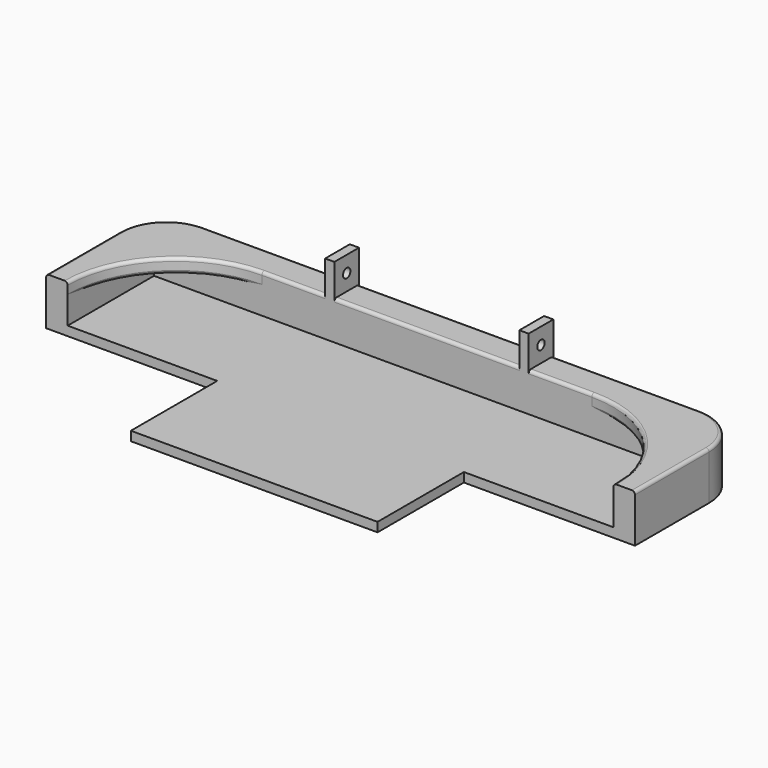
from build123d import *

# Parameters (mm, degrees)
F0_W         = 80
F0_H         = 35
F0_W_2       = 60
F0_H_2       = 10
F0_W_3       = 3
F1_DEPTH     = 3
F2_DEPTH     = 12.525
F3_DEPTH     = 7.968
F4_DEPTH     = 23
F5_R         = 1.5
F6_DEPTH     = 128.501
F7_T1_DEPTH  = 60
F7_T3_DEPTH  = 47.5
F7_T5_DEPTH  = 20.5
F7_T7_DEPTH  = 32.5
F7_T9_DEPTH  = 20.5
F7_T11_DEPTH = 47.5
F7_T16_ANGLE = 130.941996925
F7_T22_ANGLE = 130.941996925
F7_T26_ANGLE = 94.0941996925
F7_T28_ANGLE = 94.0941996925
F7_T30_ANGLE = 90
F7_T32_ANGLE = 90


# Not quite as in the source:
# - a fillet or chamfer that OpenCascade refuses, or shapes differently, is made with other operations: its cross-section is extruded or revolved along the edge and cut away or added


with BuildPart() as f1:
    # F0 (on Top) → F1 (new body)
    with BuildSketch(Plane.XY):
        with Locations((0, -17.5)):
            Rectangle(F0_W, F0_H)
        with BuildLine():
            Line((-88.5, 35), (-88.5, 0))
            ThreePointArc((-88.5, 0), (-78.2487373415, 24.7487373415), (-53.5, 35))
            Line((-53.5, 35), (-88.5, 35))
        make_face()
        with BuildLine():
            ThreePointArc((53.5, 35), (78.2487373415, 24.7487373415), (88.5, 0))
            Line((88.5, 0), (88.5, 35))
            Line((88.5, 35), (53.5, 35))
        make_face()
        with BuildLine():
            Line((-95.5, 30), (-95.5, 0))
            Line((-95.5, 0), (-88.5, 0))
            Line((-88.5, 0), (-88.5, 35))
            Line((-88.5, 35), (-53.5, 35))
            Line((-53.5, 35), (-33, 35))
            Line((-33, 35), (-33, 45))
            Line((-33, 45), (-80.5, 45))
            ThreePointArc((-80.5, 45), (-91.1066017178, 40.6066017178), (-95.5, 30))
        make_face()
        with Locations((0, 40)):
            Rectangle(F0_W_2, F0_H_2)
        with BuildLine():
            Line((88.5, 35), (88.5, 0))
            Line((88.5, 0), (95.5, 0))
            Line((95.5, 0), (95.5, 30))
            ThreePointArc((95.5, 30), (91.1066017178, 40.6066017178), (80.5, 45))
            Line((80.5, 45), (33, 45))
            Line((33, 45), (33, 35))
            Line((33, 35), (53.5, 35))
            Line((53.5, 35), (88.5, 35))
        make_face()
        with Locations((-31.5, 40)):
            Rectangle(F0_W_3, F0_H_2)
        with Locations((31.5, 40)):
            Rectangle(F0_W_3, F0_H_2)
        with BuildLine():
            ThreePointArc((-53.5, 35), (-78.2487373415, 24.7487373415), (-88.5, 0))
            Line((-88.5, 0), (-40, 0))
            Line((-40, 0), (40, 0))
            Line((40, 0), (88.5, 0))
            ThreePointArc((88.5, 0), (78.2487373415, 24.7487373415), (53.5, 35))
            Line((53.5, 35), (33, 35))
            Line((33, 35), (30, 35))
            Line((30, 35), (-30, 35))
            Line((-30, 35), (-33, 35))
            Line((-33, 35), (-53.5, 35))
        make_face()
    extrude(amount=-F1_DEPTH)

    # F0 (on Top) → F2 (join)
    with BuildSketch(Plane.XY):
        with BuildLine():
            Line((-95.5, 30), (-95.5, 0))
            Line((-95.5, 0), (-88.5, 0))
            Line((-88.5, 0), (-88.5, 35))
            Line((-88.5, 35), (-53.5, 35))
            Line((-53.5, 35), (-33, 35))
            Line((-33, 35), (-33, 45))
            Line((-33, 45), (-80.5, 45))
            ThreePointArc((-80.5, 45), (-91.1066017178, 40.6066017178), (-95.5, 30))
        make_face()
        with Locations((-31.5, 40)):
            Rectangle(F0_W_3, F0_H_2)
        with Locations((0, 40)):
            Rectangle(F0_W_2, F0_H_2)
        with Locations((31.5, 40)):
            Rectangle(F0_W_3, F0_H_2)
        with BuildLine():
            Line((88.5, 35), (88.5, 0))
            Line((88.5, 0), (95.5, 0))
            Line((95.5, 0), (95.5, 30))
            ThreePointArc((95.5, 30), (91.1066017178, 40.6066017178), (80.5, 45))
            Line((80.5, 45), (33, 45))
            Line((33, 45), (33, 35))
            Line((33, 35), (53.5, 35))
            Line((53.5, 35), (88.5, 35))
        make_face()
        with BuildLine():
            Line((-88.5, 35), (-88.5, 0))
            ThreePointArc((-88.5, 0), (-78.2487373415, 24.7487373415), (-53.5, 35))
            Line((-53.5, 35), (-88.5, 35))
        make_face()
        with BuildLine():
            ThreePointArc((53.5, 35), (78.2487373415, 24.7487373415), (88.5, 0))
            Line((88.5, 0), (88.5, 35))
            Line((88.5, 35), (53.5, 35))
        make_face()
    extrude(amount=F2_DEPTH)

    # F0 (on Top) → F3 (cut)
    with BuildSketch(Plane.XY):
        with BuildLine():
            Line((-88.5, 35), (-88.5, 0))
            ThreePointArc((-88.5, 0), (-78.2487373415, 24.7487373415), (-53.5, 35))
            Line((-53.5, 35), (-88.5, 35))
        make_face()
        with BuildLine():
            ThreePointArc((53.5, 35), (78.2487373415, 24.7487373415), (88.5, 0))
            Line((88.5, 0), (88.5, 35))
            Line((88.5, 35), (53.5, 35))
        make_face()
    extrude(amount=F3_DEPTH, mode=Mode.SUBTRACT)

    # F0 (on Top) → F4 (join)
    with BuildSketch(Plane.XY):
        with Locations((-31.5, 40)):
            Rectangle(F0_W_3, F0_H_2)
        with Locations((31.5, 40)):
            Rectangle(F0_W_3, F0_H_2)
    extrude(amount=F4_DEPTH)

    # F5 (on face) → F6 (cut, through all)
    with BuildSketch(Plane(origin=(-33, 0, 0), x_dir=(0, -1, 0), z_dir=(-1, 0, 0))):
        with Locations((-40, 17.7625)):
            Circle(F5_R)
    extrude(amount=-F6_DEPTH, mode=Mode.SUBTRACT)

    # F7: fillet of radius 1 on 14 edges, made by hand

    # F7_s2 → F7_t1 (cut)
    with BuildSketch(Plane.YZ.offset(-30)):
        with BuildLine():
            ThreePointArc((45, 11.525), (44.7071067812, 12.2321067812), (44, 12.525))
            Line((44, 12.525), (45, 12.525))
            Line((45, 12.525), (45, 11.525))
        make_face()
        with BuildLine():
            ThreePointArc((35, 11.525), (35.2928932188, 12.2321067812), (36, 12.525))
            Line((36, 12.525), (35, 12.525))
            Line((35, 12.525), (35, 11.525))
        make_face()
    extrude(amount=F7_T1_DEPTH, mode=Mode.SUBTRACT)

    # F7_s4 → F7_t3 (cut)
    with BuildSketch(Plane.YZ.offset(-80.5)):
        with BuildLine():
            ThreePointArc((44, 12.525), (44.7071067812, 12.2321067812), (45, 11.525))
            Line((45, 11.525), (45, 12.525))
            Line((45, 12.525), (44, 12.525))
        make_face()
    extrude(amount=F7_T3_DEPTH, mode=Mode.SUBTRACT)

    # F7_s6 → F7_t5 (cut)
    with BuildSketch(Plane.YZ.offset(-53.5)):
        with BuildLine():
            ThreePointArc((36, 12.525), (35.2928932188, 12.2321067812), (35, 11.525))
            Line((35, 11.525), (35, 12.525))
            Line((35, 12.525), (36, 12.525))
        make_face()
    extrude(amount=F7_T5_DEPTH, mode=Mode.SUBTRACT)

    # F7_s8 → F7_t7 (cut)
    with BuildSketch(Plane.XZ.offset(-30)):
        with BuildLine():
            ThreePointArc((-94.5, 12.525), (-95.2071067812, 12.2321067812), (-95.5, 11.525))
            Line((-95.5, 11.525), (-95.5, 12.525))
            Line((-95.5, 12.525), (-94.5, 12.525))
        make_face()
        with BuildLine():
            ThreePointArc((95.5, 11.525), (95.2071067812, 12.2321067812), (94.5, 12.525))
            Line((94.5, 12.525), (95.5, 12.525))
            Line((95.5, 12.525), (95.5, 11.525))
        make_face()
    extrude(amount=F7_T7_DEPTH, mode=Mode.SUBTRACT)

    # F7_s10 → F7_t9 (cut)
    with BuildSketch(Plane.YZ.offset(33)):
        with BuildLine():
            ThreePointArc((35, 11.525), (35.2928932188, 12.2321067812), (36, 12.525))
            Line((36, 12.525), (35, 12.525))
            Line((35, 12.525), (35, 11.525))
        make_face()
    extrude(amount=F7_T9_DEPTH, mode=Mode.SUBTRACT)

    # F7_s12 → F7_t11 (cut)
    with BuildSketch(Plane.YZ.offset(33)):
        with BuildLine():
            ThreePointArc((45, 11.525), (44.7071067812, 12.2321067812), (44, 12.525))
            Line((44, 12.525), (45, 12.525))
            Line((45, 12.525), (45, 11.525))
        make_face()
    extrude(amount=F7_T11_DEPTH, mode=Mode.SUBTRACT)


with BuildPart() as f7_tool14:
    # F7_s15 → F7_t16 (revolve)
    with BuildSketch(Plane(origin=(-6.5437628549, 17.5291323355, 0), x_dir=(0, 0, 1), z_dir=(0.3497332189, -0.9368493345, 0))):
        with BuildLine():
            ThreePointArc((8.968, 85.1214393974), (8.2608932188, 85.4143326162), (7.968, 86.1214393974))
            Line((7.968, 86.1214393974), (7.968, 85.1214393974))
            Line((7.968, 85.1214393974), (8.968, 85.1214393974))
        make_face()
    revolve(axis=Axis((-53.5, 0, 7.968), (0, 0, -1)), revolution_arc=F7_T16_ANGLE)

    split(bisect_by=Plane.YZ.offset(-88.5), keep=Keep.TOP)

    split(bisect_by=Plane.XZ.offset(-35), keep=Keep.TOP)


with BuildPart() as f1_1:
    add(f1.part)

    # F7_t13: cut F7_tool14
    add(f7_tool14.part, mode=Mode.SUBTRACT)


with BuildPart() as f7_tool20:
    # F7_s21 → F7_t22 (revolve)
    with BuildSketch(Plane(origin=(46.9562371451, 17.5291323355, 0), x_dir=(0, 0, 1), z_dir=(-0.9368493345, -0.3497332189, 0))):
        with BuildLine():
            ThreePointArc((8.968, 16.2892727897), (8.2608932188, 16.5821660086), (7.968, 17.2892727897))
            Line((7.968, 17.2892727897), (7.968, 16.2892727897))
            Line((7.968, 16.2892727897), (8.968, 16.2892727897))
        make_face()
    revolve(axis=Axis((53.5, 0, 7.968), (0, 0, -1)), revolution_arc=F7_T22_ANGLE)

    split(bisect_by=Plane.YZ.offset(88.5), keep=Keep.BOTTOM)

    split(bisect_by=Plane.XZ.offset(-35), keep=Keep.TOP)


with BuildPart() as f1_2:
    add(f1_1.part)

    # F7_t19: cut F7_tool20
    add(f7_tool20.part, mode=Mode.SUBTRACT)

    # F7_s25 → F7_t26 (revolve, cut)
    with BuildSketch(Plane(origin=(-0.2727138814, 3.809963227, 0), x_dir=(0, 0, 1), z_dir=(0.0713964686, -0.9974480158, 0))):
        with BuildLine():
            ThreePointArc((11.525, 88.3634688467), (12.2321067812, 88.6563620655), (12.525, 89.3634688467))
            Line((12.525, 89.3634688467), (12.525, 88.3634688467))
            Line((12.525, 88.3634688467), (11.525, 88.3634688467))
        make_face()
    revolve(axis=Axis((-53.5, 0, 12.525), (0, 0, -1)), revolution_arc=F7_T26_ANGLE, mode=Mode.SUBTRACT)

    # F7_s27 → F7_t28 (revolve, cut)
    with BuildSketch(Plane.YZ.offset(53.5)):
        with BuildLine():
            ThreePointArc((36, 12.525), (35.2928932188, 12.2321067812), (35, 11.525))
            Line((35, 11.525), (35, 12.525))
            Line((35, 12.525), (36, 12.525))
        make_face()
    revolve(axis=Axis((53.5, 0, 12.525), (0, 0, -1)), revolution_arc=F7_T28_ANGLE, mode=Mode.SUBTRACT)

    # F7_s29 → F7_t30 (revolve, cut)
    with BuildSketch(Plane.XZ.offset(-30)):
        with BuildLine():
            ThreePointArc((95.5, 11.525), (95.2071067812, 12.2321067812), (94.5, 12.525))
            Line((94.5, 12.525), (95.5, 12.525))
            Line((95.5, 12.525), (95.5, 11.525))
        make_face()
    revolve(axis=Axis((80.5, 30, 12.525), (0, 0, 1)), revolution_arc=F7_T30_ANGLE, mode=Mode.SUBTRACT)

    # F7_s31 → F7_t32 (revolve, cut)
    with BuildSketch(Plane.YZ.offset(-80.5)):
        with BuildLine():
            ThreePointArc((44, 12.525), (44.7071067812, 12.2321067812), (45, 11.525))
            Line((45, 11.525), (45, 12.525))
            Line((45, 12.525), (44, 12.525))
        make_face()
    revolve(axis=Axis((-80.5, 30, 12.525), (0, 0, 1)), revolution_arc=F7_T32_ANGLE, mode=Mode.SUBTRACT)


solid = f1_2.part
